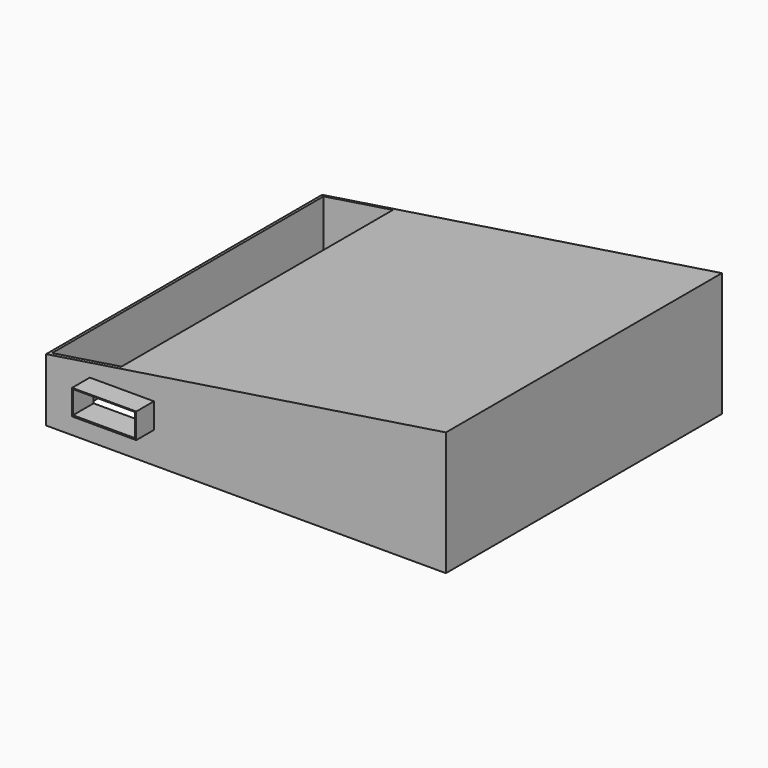
from build123d import *

# Parameters (mm, degrees)
F0_W      = 5686.5700594
F0_H      = 4907.2993548
F2_DEPTH  = 1051.56
F3_W      = 912.28556633
F3_H      = 358.6589396
F4_DEPTH  = 314.96
F5_W      = 883.4848403931
F5_H      = 326.3165652752
F6_DEPTH  = 1803.4
F7_W      = 5686.5700594
F7_H      = 4907.2993548
F8_DEPTH  = 711.2
F10_DEPTH = 6418.58


# Not quite as in the source:
# - the program builds the solid bodies; features that only make, move or delete a surface that nothing else refers to are left out


with BuildPart() as f2:
    # F0 (on Top) → F2 (new body)
    with BuildSketch(Plane.XY):
        with Locations((-1.27e-05, 0)):
            Rectangle(F0_W, F0_H)
        Polygon((-2798.8430942, 1200.4981324), (-2798.8430942, 2423.930382), (-1600.664185, 2423.930382), (-1528.8430942, 2423.930382), (2789.1569058, 2423.930382), (2789.1569058, -2402.069618), (-2798.8430942, -2402.069618), (-2798.8430942, 1128.530382), align=None, mode=Mode.SUBTRACT)
    extrude(amount=F2_DEPTH)

    # F3 (on face) → F4 (join)
    with BuildSketch(Plane.XZ.offset(2453.6496774)):
        with Locations((-1765.2000188828, 623.0345219374)):
            Rectangle(F3_W, F3_H)
    extrude(amount=F4_DEPTH)

    # F5 (on face) → F6 (cut)
    with BuildSketch(Plane.XZ.offset(2768.6096774)):
        with Locations((-1766.7844295502, 626.5381127596)):
            Rectangle(F5_W, F5_H)
    extrude(amount=-F6_DEPTH, mode=Mode.SUBTRACT)

    # F7 (on face) → F8 (join)
    with BuildSketch(Plane.XY.offset(1051.56)):
        with Locations((-1.27e-05, 0)):
            Rectangle(F7_W, F7_H)
    extrude(amount=F8_DEPTH)

    # F9 (on face) → F10 (cut)
    with BuildSketch(Plane.XZ.offset(2453.6496774)):
        Polygon((-2843.2850424, 1762.76), (-2843.2850424, 894.1189227129), (2843.285017, 1762.76), align=None)
    extrude(amount=-F10_DEPTH, mode=Mode.SUBTRACT)


solid = f2.part
